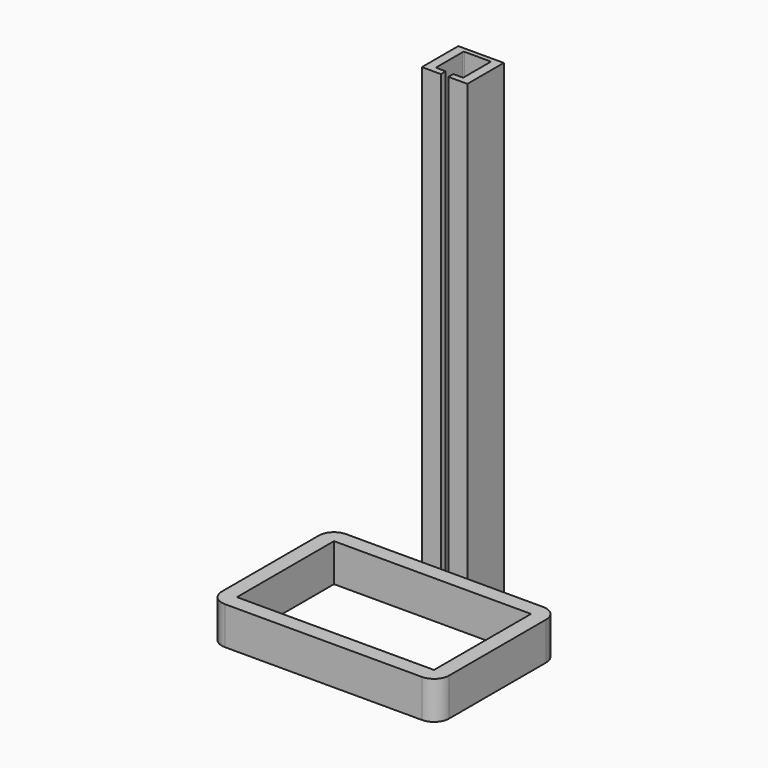
from build123d import *

# Parameters (mm, degrees)
F1_DEPTH      = 12.5
F2_DEPTH      = 300
F2_DEPTH_BACK = 12.5
F0_R          = 6
F3_DEPTH      = 50
F4_R          = 0.5


# Not quite as in the source:
# - a feature names something its author has since deleted; it is built from what else it names


with BuildPart() as f1:
    # F0 (on Top) → F1 (new body, symmetric)
    with BuildSketch(Plane.XY):
        with BuildLine():
            Line((-15, 50), (-65, 50))
            ThreePointArc((-65, 50), (-72.0710678119, 47.0710678119), (-75, 40))
            Line((-75, 40), (-75, -40))
            ThreePointArc((-75, -40), (-72.0710678119, -47.0710678119), (-65, -50))
            Line((-65, -50), (65, -50))
            ThreePointArc((65, -50), (72.0710678119, -47.0710678119), (75, -40))
            Line((75, -40), (75, 40))
            ThreePointArc((75, 40), (72.0710678119, 47.0710678119), (65, 50))
            Line((65, 50), (15, 50))
            Line((15, 50), (2.5, 50))
            Line((2.5, 50), (2.5, 40.0037090484))
            Line((2.5, 40.0037090484), (65, 40.0037090484))
            Line((65, 40.0037090484), (65, -40.0037090484))
            Line((65, -40.0037090484), (-65, -40.0037090484))
            Line((-65, -40.0037090484), (-65, 40.0037090484))
            Line((-65, 40.0037090484), (-2.5, 40.0037090484))
            Line((-2.5, 40.0037090484), (-2.5, 50))
            Line((-2.5, 50), (-15, 50))
        make_face()
        Polygon((2.5, 50), (-2.5, 50), (-2.5, 40.0037090484), (0, 40.0037090484), (2.5, 40.0037090484), align=None)
    extrude(amount=F1_DEPTH, both=True)

    # F0 (on Top) → F2 (join, two sides)
    with BuildSketch(Plane.XY) as f2_sk:
        Polygon((-15, 80), (-15, 50), (-2.5, 50), (-2.5, 53.9933157269), (-9, 53.9933157269), (-9, 76.9933157269), (0, 76.9933157269), (0, 79.2549662558), (0, 80), align=None)
        Polygon((2.5, 53.9933157269), (2.5, 50), (15, 50), (15, 80), (0, 80), (0, 79.2549662558), (0, 76.9933157269), (9, 76.9933157269), (9, 53.9933157269), align=None)
    extrude(amount=F2_DEPTH)
    extrude(f2_sk.sketch, amount=-F2_DEPTH_BACK)

    # F0 (on Top) → F3 (cut)
    with BuildSketch(Plane.XY):
        with Locations((0, 69.7)):
            Circle(F0_R)
    extrude(amount=F3_DEPTH, mode=Mode.SUBTRACT)

    # F4
    f4_edges = [f1.edges().sort_by_distance(p)[0] for p in [
        (-9, 76.993316, 143.75),
        (9, 76.993316, 143.75),
        (-9, 53.993316, 143.75),
        (9, 53.993316, 143.75),
    ]]
    fillet(f4_edges, radius=F4_R)


solid = f1.part
